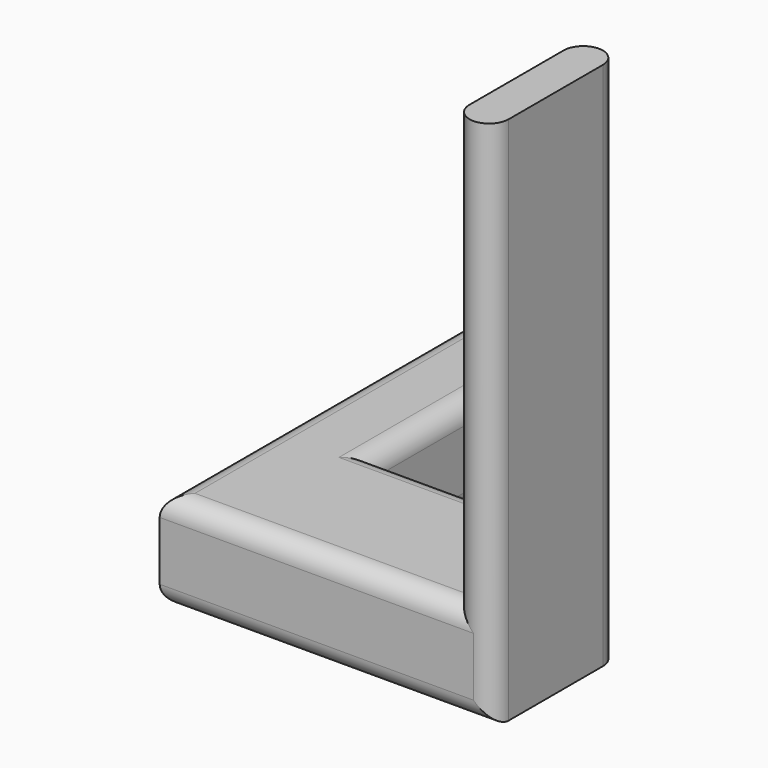
from build123d import *

# Parameters (mm, degrees)
F0_W         = 70
F0_H         = 40
F0_W_2       = 15
F1_DEPTH     = 25
F2_W         = 10
F2_H         = 40
F3_DEPTH     = 110
F4_W         = 22.7000065148
F4_H         = 25
F5_DEPTH     = 70
F6_R         = 14.75
F7_DEPTH     = 5
F8_T1_DEPTH  = 87.5
F8_T3_DEPTH  = 52.2999934852
F8_T5_DEPTH  = 82.5
F8_T7_DEPTH  = 135
F8_T9_DEPTH  = 110
F8_T11_DEPTH = 160
F8_T13_DEPTH = 122.5
F8_T19_DEPTH = 100
F8_T23_DEPTH = 135
F8_T30_DEPTH = 64.7999934852
F8_T34_DEPTH = 135
F8_T41_DEPTH = 64.7999934852
F8_T45_DEPTH = 95


# Not quite as in the source:
# - a fillet or chamfer that OpenCascade refuses, or shapes differently, is made with other operations: its cross-section is extruded or revolved along the edge and cut away or added


with BuildPart() as f1:
    # F0 (on Top) → F1 (new body)
    with BuildSketch(Plane.XY):
        with Locations((-33.8003174961, 0.9457613719)):
            Rectangle(F0_W, F0_H)
        with Locations((8.6996825039, 0.9457613719)):
            Rectangle(F0_W_2, F0_H)
    extrude(amount=F1_DEPTH)

    # F2 (on face) → F3 (join)
    with BuildSketch(Plane.XY.offset(25)):
        with Locations((11.1996825039, 0.9457613719)):
            Rectangle(F2_W, F2_H)
    extrude(amount=F3_DEPTH)

    # F4 (on face) → F5 (join)
    with BuildSketch(Plane(origin=(0, 20.9457613719, 0), x_dir=(-1, 0, 0), z_dir=(0, 1, 0))):
        with Locations((57.4503142387, 12.5)):
            Rectangle(F4_W, F4_H)
    extrude(amount=F5_DEPTH)

    # F6 (on face) → F7 (cut)
    with BuildSketch(Plane(origin=(6.1996825039, 0, 0), x_dir=(0, -1, 0), z_dir=(-1, 0, 0))):
        with Locations((0, 108.7849736214)):
            Circle(F6_R)
    extrude(amount=-F7_DEPTH, mode=Mode.SUBTRACT)

    # F8: fillet of radius 5 on 11 edges, made by hand

    # F8_s2 → F8_t1 (cut)
    with BuildSketch(Plane.YZ.offset(-81.3003174961)):
        with BuildLine():
            ThreePointArc((-19.0542386281, 20), (-17.589772534, 23.5355339059), (-14.0542386281, 25))
            Line((-14.0542386281, 25), (-19.0542386281, 25))
            Line((-19.0542386281, 25), (-19.0542386281, 20))
        make_face()
    extrude(amount=F8_T1_DEPTH, mode=Mode.SUBTRACT)

    # F8_s4 → F8_t3 (cut)
    with BuildSketch(Plane.YZ.offset(-46.1003109813)):
        with BuildLine():
            ThreePointArc((15.9457613719, 25), (19.4812952778, 23.5355339059), (20.9457613719, 20))
            Line((20.9457613719, 20), (20.9457613719, 25))
            Line((20.9457613719, 25), (15.9457613719, 25))
        make_face()
    extrude(amount=F8_T3_DEPTH, mode=Mode.SUBTRACT)

    # F8_s6 → F8_t5 (cut)
    with BuildSketch(Plane.XZ.offset(-103.4457613719)):
        with BuildLine():
            ThreePointArc((-51.1003109813, 25), (-47.5647770753, 23.5355339059), (-46.1003109813, 20))
            Line((-46.1003109813, 20), (-46.1003109813, 25))
            Line((-46.1003109813, 25), (-51.1003109813, 25))
        make_face()
        with BuildLine():
            ThreePointArc((-51.1003109813, 0), (-47.5647770753, 1.4644660941), (-46.1003109813, 5))
            Line((-46.1003109813, 5), (-46.1003109813, 0))
            Line((-46.1003109813, 0), (-51.1003109813, 0))
        make_face()
    extrude(amount=F8_T5_DEPTH, mode=Mode.SUBTRACT)

    # F8_s8 → F8_t7 (cut)
    with BuildSketch(Plane.XZ.offset(-103.4457613719)):
        with BuildLine():
            ThreePointArc((-68.8003174961, 20), (-67.335851402, 23.5355339059), (-63.8003174961, 25))
            Line((-63.8003174961, 25), (-68.8003174961, 25))
            Line((-68.8003174961, 25), (-68.8003174961, 20))
        make_face()
        with BuildLine():
            ThreePointArc((-68.8003174961, 5), (-67.335851402, 1.4644660941), (-63.8003174961, 0))
            Line((-63.8003174961, 0), (-68.8003174961, 0))
            Line((-68.8003174961, 0), (-68.8003174961, 5))
        make_face()
    extrude(amount=F8_T7_DEPTH, mode=Mode.SUBTRACT)

    # F8_s10 → F8_t9 (cut)
    with BuildSketch(Plane.YZ.offset(-81.3003174961)):
        with BuildLine():
            ThreePointArc((-19.0542386281, 5), (-17.589772534, 1.4644660941), (-14.0542386281, 0))
            Line((-14.0542386281, 0), (-19.0542386281, 0))
            Line((-19.0542386281, 0), (-19.0542386281, 5))
        make_face()
    extrude(amount=F8_T9_DEPTH, mode=Mode.SUBTRACT)

    # F8_s12 → F8_t11 (cut)
    with BuildSketch(Plane.XY.offset(-12.5)):
        with BuildLine():
            ThreePointArc((11.1996825039, -19.0542386281), (14.7352164099, -17.589772534), (16.1996825039, -14.0542386281))
            Line((16.1996825039, -14.0542386281), (16.1996825039, -19.0542386281))
            Line((16.1996825039, -19.0542386281), (11.1996825039, -19.0542386281))
        make_face()
        with BuildLine():
            ThreePointArc((16.1996825039, 15.9457613719), (14.7352164099, 19.4812952778), (11.1996825039, 20.9457613719))
            Line((11.1996825039, 20.9457613719), (16.1996825039, 20.9457613719))
            Line((16.1996825039, 20.9457613719), (16.1996825039, 15.9457613719))
        make_face()
    extrude(amount=F8_T11_DEPTH, mode=Mode.SUBTRACT)

    # F8_s14 → F8_t13 (cut)
    with BuildSketch(Plane.XY.offset(25)):
        with BuildLine():
            ThreePointArc((11.1996825039, -19.0542386281), (7.664148598, -17.589772534), (6.1996825039, -14.0542386281))
            Line((6.1996825039, -14.0542386281), (6.1996825039, -19.0542386281))
            Line((6.1996825039, -19.0542386281), (11.1996825039, -19.0542386281))
        make_face()
        with BuildLine():
            ThreePointArc((6.1996825039, 15.9457613719), (7.664148598, 19.4812952778), (11.1996825039, 20.9457613719))
            Line((11.1996825039, 20.9457613719), (6.1996825039, 20.9457613719))
            Line((6.1996825039, 20.9457613719), (6.1996825039, 15.9457613719))
        make_face()
    extrude(amount=F8_T13_DEPTH, mode=Mode.SUBTRACT)


with BuildPart() as f8_tool17:
    # F8_s18 → F8_t19 (new body)
    with BuildSketch(Plane.YZ.offset(-81.3003174961)):
        with BuildLine():
            ThreePointArc((-19.0542386281, 20), (-17.589772534, 23.5355339059), (-14.0542386281, 25))
            Line((-14.0542386281, 25), (-19.0542386281, 25))
            Line((-19.0542386281, 25), (-19.0542386281, 20))
        make_face()
    extrude(amount=F8_T19_DEPTH)

    split(bisect_by=Plane.YZ.offset(6.1996825039), keep=Keep.TOP)


with BuildPart() as f8_tool21:
    # F8_s22 → F8_t23 (new body)
    with BuildSketch(Plane.XY.offset(12.5)):
        with BuildLine():
            ThreePointArc((11.1996825039, -19.0542386281), (7.664148598, -17.589772534), (6.1996825039, -14.0542386281))
            Line((6.1996825039, -14.0542386281), (6.1996825039, -19.0542386281))
            Line((6.1996825039, -19.0542386281), (11.1996825039, -19.0542386281))
        make_face()
    extrude(amount=F8_T23_DEPTH)

    split(bisect_by=Plane.XY.offset(25), keep=Keep.BOTTOM)


with BuildPart() as f8_tool17_1:
    add(f8_tool17.part)

    # F8_t25: intersect F8_tool21
    add(f8_tool21.part, mode=Mode.INTERSECT)


with BuildPart() as f1_1:
    add(f1.part)

    # F8_t15: cut F8_tool17
    add(f8_tool17_1.part, mode=Mode.SUBTRACT)


with BuildPart() as f8_tool28:
    # F8_s29 → F8_t30 (new body)
    with BuildSketch(Plane.YZ.offset(18.6996825039)):
        with BuildLine():
            ThreePointArc((15.9457613719, 25), (19.4812952778, 23.5355339059), (20.9457613719, 20))
            Line((20.9457613719, 20), (20.9457613719, 25))
            Line((20.9457613719, 25), (15.9457613719, 25))
        make_face()
    extrude(amount=-F8_T30_DEPTH)

    split(bisect_by=Plane.YZ.offset(6.1996825039), keep=Keep.TOP)


with BuildPart() as f8_tool32:
    # F8_s33 → F8_t34 (new body)
    with BuildSketch(Plane.XY.offset(12.5)):
        with BuildLine():
            ThreePointArc((6.1996825039, 15.9457613719), (7.664148598, 19.4812952778), (11.1996825039, 20.9457613719))
            Line((11.1996825039, 20.9457613719), (6.1996825039, 20.9457613719))
            Line((6.1996825039, 20.9457613719), (6.1996825039, 15.9457613719))
        make_face()
    extrude(amount=F8_T34_DEPTH)

    split(bisect_by=Plane.XY.offset(25), keep=Keep.BOTTOM)


with BuildPart() as f8_tool28_1:
    add(f8_tool28.part)

    # F8_t36: intersect F8_tool32
    add(f8_tool32.part, mode=Mode.INTERSECT)


with BuildPart() as f1_2:
    add(f1_1.part)

    # F8_t26: cut F8_tool28
    add(f8_tool28_1.part, mode=Mode.SUBTRACT)


with BuildPart() as f8_tool39:
    # F8_s40 → F8_t41 (new body)
    with BuildSketch(Plane.YZ.offset(6.1996825039)):
        with BuildLine():
            ThreePointArc((15.9457613719, 25), (19.4812952778, 23.5355339059), (20.9457613719, 20))
            Line((20.9457613719, 20), (20.9457613719, 25))
            Line((20.9457613719, 25), (15.9457613719, 25))
        make_face()
    extrude(amount=-F8_T41_DEPTH)

    split(bisect_by=Plane.YZ.offset(-46.1003109813), keep=Keep.BOTTOM)


with BuildPart() as f8_tool43:
    # F8_s44 → F8_t45 (new body)
    with BuildSketch(Plane.XZ.offset(-8.4457613719)):
        with BuildLine():
            ThreePointArc((-51.1003109813, 25), (-47.5647770753, 23.5355339059), (-46.1003109813, 20))
            Line((-46.1003109813, 20), (-46.1003109813, 25))
            Line((-46.1003109813, 25), (-51.1003109813, 25))
        make_face()
    extrude(amount=-F8_T45_DEPTH)

    split(bisect_by=Plane.XZ.offset(-20.9457613719), keep=Keep.TOP)


with BuildPart() as f8_tool39_1:
    add(f8_tool39.part)

    # F8_t47: intersect F8_tool43
    add(f8_tool43.part, mode=Mode.INTERSECT)


with BuildPart() as f1_3:
    add(f1_2.part)

    # F8_t37: cut F8_tool39
    add(f8_tool39_1.part, mode=Mode.SUBTRACT)


solid = f1_3.part
